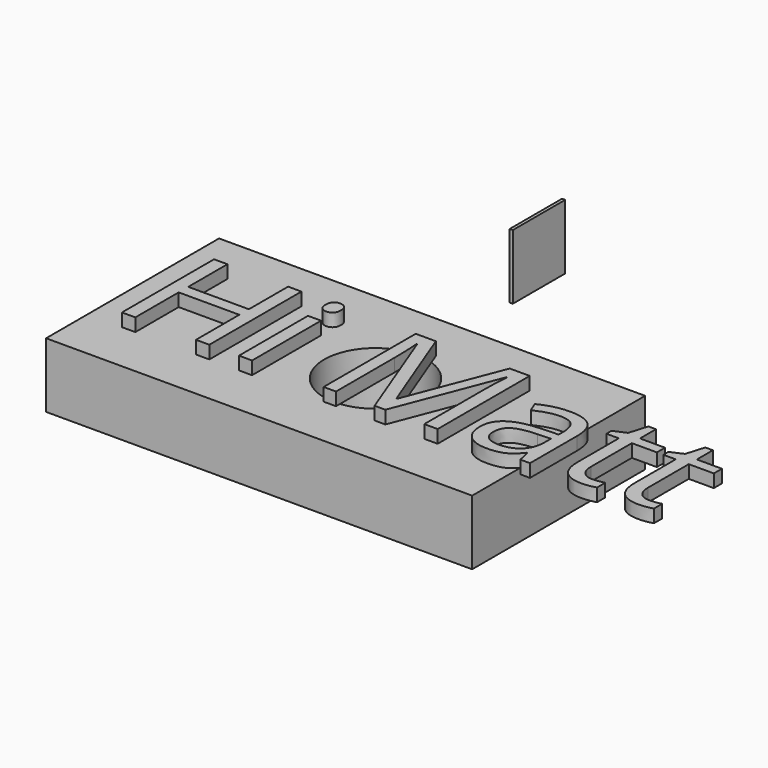
from build123d import *

# Parameters (mm, degrees)
F1_START     = 6.35
F0_W         = 83.4355382249
F0_H         = 42.3401389271
F1_DEPTH     = 12.7
F0_W_2       = 0.6130076945
F0_H_2       = 12.8312036395
F2_R         = 10.0554490687
F3_DEPTH     = 12.7
F4_TEXT_SIZE = 31.5779871825
F5_DEPTH     = 2.54


# Not quite as in the source:
# - Text() gives the source's letters only with a copy of the font that has no kerning and outlines rounded to 1/6400 em; it was checked with that copy


with BuildPart() as f1:
    # F0 (on Top) → F1 (new body)
    with BuildSketch(Plane.XY.offset(F1_START)):
        with Locations((53.4479753114, 36.2036405131)):
            Rectangle(F0_W, F0_H)
    extrude(amount=F1_DEPTH)

    # F2 (on face) → F3 (cut, through all)
    with BuildSketch(Plane.XY.offset(19.05)):
        with Locations((59.3756847084, 36.1166708171)):
            Circle(F2_R)
    extrude(amount=-F3_DEPTH, mode=Mode.SUBTRACT)

    # F4 (on face) → F5 (join)
    with BuildSketch(Plane.XY.offset(19.05)):
        with Locations((15.3997214511, 25.1449011266)):
            Text('Hi Matt', F4_TEXT_SIZE, font='Open Sans', text_align=(TextAlign.LEFT, TextAlign.BOTTOM))
    extrude(amount=F5_DEPTH)


with BuildPart() as f1b:
    # F0 (on Top) → F1, piece 2 (new body)
    with BuildSketch(Plane.XY.offset(F1_START)):
        with Locations((44.7793137282, 93.9945913851)):
            Rectangle(F0_W_2, F0_H_2)
    extrude(amount=F1_DEPTH)


solid = Compound([f1.part, f1b.part])
